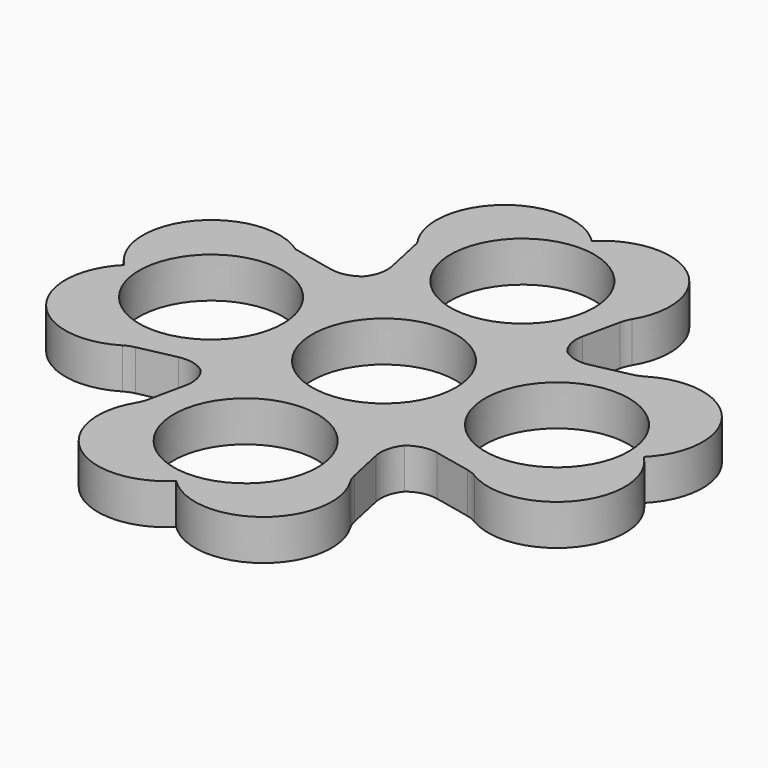
from build123d import *

# Parameters (mm, degrees)
F0_R        = 11.2522
F1_DEPTH    = 6.35
F2_T1_DEPTH = 6.35


# Not quite as in the source:
# - a fillet or chamfer that OpenCascade refuses, or shapes differently, is made with other operations: its cross-section is extruded or revolved along the edge and cut away or added


with BuildPart() as f1:
    # F0 (on Top) → F1 (new body)
    with BuildSketch(Plane.XY):
        with BuildLine():
            Line((-16.3332085084, 26.9033375639), (-14.2845390508, 17.386659874))
            ThreePointArc((-14.2845390508, 17.386659874), (-15.9113795359, 15.9113795359), (-17.386659874, 14.2845390508))
            Line((-17.386659874, 14.2845390508), (-26.9033375639, 16.3332085084))
            ThreePointArc((-26.9033375639, 16.3332085084), (-41.2837315607, 14.4844486959), (-40.64, 0))
            ThreePointArc((-40.64, 0), (-41.2837315607, -14.4844486959), (-26.9033375639, -16.3332085084))
            Line((-26.9033375639, -16.3332085084), (-17.386659874, -14.2845390508))
            ThreePointArc((-17.386659874, -14.2845390508), (-15.9113795359, -15.9113795359), (-14.2845390508, -17.386659874))
            Line((-14.2845390508, -17.386659874), (-16.3332085084, -26.9033375639))
            ThreePointArc((-16.3332085084, -26.9033375639), (-14.4844486959, -41.2837315607), (0, -40.64))
            ThreePointArc((0, -40.64), (14.4844486959, -41.2837315607), (16.3332085084, -26.9033375639))
            Line((16.3332085084, -26.9033375639), (14.2845390508, -17.386659874))
            ThreePointArc((14.2845390508, -17.386659874), (15.9113795359, -15.9113795359), (17.386659874, -14.2845390508))
            Line((17.386659874, -14.2845390508), (26.9033375639, -16.3332085084))
            ThreePointArc((26.9033375639, -16.3332085084), (41.2837315607, -14.4844486959), (40.64, 0))
            ThreePointArc((40.64, 0), (41.2837315607, 14.4844486959), (26.9033375639, 16.3332085084))
            Line((26.9033375639, 16.3332085084), (17.386659874, 14.2845390508))
            ThreePointArc((17.386659874, 14.2845390508), (15.9113795359, 15.9113795359), (14.2845390508, 17.386659874))
            Line((14.2845390508, 17.386659874), (16.3332085084, 26.9033375639))
            ThreePointArc((16.3332085084, 26.9033375639), (14.4844486959, 41.2837315607), (0, 40.64))
            ThreePointArc((0, 40.64), (-14.4844486959, 41.2837315607), (-16.3332085084, 26.9033375639))
        make_face()
        with Locations((0, -27.0631238818)):
            Circle(F0_R, mode=Mode.SUBTRACT)
        with Locations((-27.0631238818, 0)):
            Circle(F0_R, mode=Mode.SUBTRACT)
        Circle(F0_R, mode=Mode.SUBTRACT)
        with Locations((27.0631238818, 0)):
            Circle(F0_R, mode=Mode.SUBTRACT)
        with Locations((0, 27.0631238818)):
            Circle(F0_R, mode=Mode.SUBTRACT)
    extrude(amount=F1_DEPTH)

    # F2: fillet of radius 5.08 on 14 edges, made by hand

    # F2_s2 → F2_t1 (join)
    with BuildSketch(Plane.XY):
        with BuildLine():
            ThreePointArc((-15.61619491, 16.2011868084), (-17.7500326172, 14.9730442969), (-20.2107454114, 14.8924841735))
            Line((-20.2107454114, 14.8924841735), (-17.386659874, 14.2845390508))
            ThreePointArc((-17.386659874, 14.2845390508), (-16.5292313987, 15.2685463237), (-15.61619491, 16.2011868084))
        make_face()
        with BuildLine():
            ThreePointArc((-14.8924841735, 20.2107454114), (-14.9730442969, 17.7500326172), (-16.2011868084, 15.61619491))
            ThreePointArc((-16.2011868084, 15.61619491), (-15.2685463237, 16.5292313987), (-14.2845390508, 17.386659874))
            Line((-14.2845390508, 17.386659874), (-14.8924841735, 20.2107454114))
        make_face()
        with BuildLine():
            ThreePointArc((20.2107454114, -14.8924841735), (17.7500326172, -14.9730442969), (15.61619491, -16.2011868084))
            ThreePointArc((15.61619491, -16.2011868084), (16.5292313987, -15.2685463237), (17.386659874, -14.2845390508))
            Line((17.386659874, -14.2845390508), (20.2107454114, -14.8924841735))
        make_face()
        with BuildLine():
            ThreePointArc((25.9885821775, -16.1362877465), (26.7940259506, -16.3810221446), (27.5479957457, -16.7554071673))
            ThreePointArc((27.5479957457, -16.7554071673), (27.221867498, -16.5501087977), (26.9033375639, -16.3332085084))
            Line((26.9033375639, -16.3332085084), (25.9885821775, -16.1362877465))
        make_face()
        with BuildLine():
            ThreePointArc((27.5479957457, 16.7554071673), (26.7940259506, 16.3810221446), (25.9885821775, 16.1362877465))
            Line((25.9885821775, 16.1362877465), (26.9033375639, 16.3332085084))
            ThreePointArc((26.9033375639, 16.3332085084), (27.221867498, 16.5501087977), (27.5479957457, 16.7554071673))
        make_face()
        with BuildLine():
            ThreePointArc((20.2107454114, 14.8924841735), (17.7500326172, 14.9730442969), (15.61619491, 16.2011868084))
            ThreePointArc((15.61619491, 16.2011868084), (16.5292313987, 15.2685463237), (17.386659874, 14.2845390508))
            Line((17.386659874, 14.2845390508), (20.2107454114, 14.8924841735))
        make_face()
        with BuildLine():
            ThreePointArc((16.2011868084, 15.61619491), (14.9730442969, 17.7500326172), (14.8924841735, 20.2107454114))
            Line((14.8924841735, 20.2107454114), (14.2845390508, 17.386659874))
            ThreePointArc((14.2845390508, 17.386659874), (15.2685463237, 16.5292313987), (16.2011868084, 15.61619491))
        make_face()
        with BuildLine():
            ThreePointArc((16.1362877465, 25.9885821775), (16.3810221446, 26.7940259506), (16.7554071673, 27.5479957457))
            ThreePointArc((16.7554071673, 27.5479957457), (16.5501087977, 27.221867498), (16.3332085084, 26.9033375639))
            Line((16.3332085084, 26.9033375639), (16.1362877465, 25.9885821775))
        make_face()
        with BuildLine():
            ThreePointArc((-27.5479957457, -16.7554071673), (-26.7940259506, -16.3810221446), (-25.9885821775, -16.1362877465))
            Line((-25.9885821775, -16.1362877465), (-26.9033375639, -16.3332085084))
            ThreePointArc((-26.9033375639, -16.3332085084), (-27.221867498, -16.5501087977), (-27.5479957457, -16.7554071673))
        make_face()
        with BuildLine():
            ThreePointArc((-20.2107454114, -14.8924841735), (-17.7500326172, -14.9730442969), (-15.61619491, -16.2011868084))
            ThreePointArc((-15.61619491, -16.2011868084), (-16.5292313987, -15.2685463237), (-17.386659874, -14.2845390508))
            Line((-17.386659874, -14.2845390508), (-20.2107454114, -14.8924841735))
        make_face()
        with BuildLine():
            ThreePointArc((-16.2011868084, -15.61619491), (-14.9730442969, -17.7500326172), (-14.8924841735, -20.2107454114))
            Line((-14.8924841735, -20.2107454114), (-14.2845390508, -17.386659874))
            ThreePointArc((-14.2845390508, -17.386659874), (-15.2685463237, -16.5292313987), (-16.2011868084, -15.61619491))
        make_face()
        with BuildLine():
            ThreePointArc((-16.1362877465, -25.9885821775), (-16.3810221446, -26.7940259506), (-16.7554071673, -27.5479957457))
            ThreePointArc((-16.7554071673, -27.5479957457), (-16.5501087977, -27.221867498), (-16.3332085084, -26.9033375639))
            Line((-16.3332085084, -26.9033375639), (-16.1362877465, -25.9885821775))
        make_face()
        with BuildLine():
            ThreePointArc((16.7554071673, -27.5479957457), (16.3810221446, -26.7940259506), (16.1362877465, -25.9885821775))
            Line((16.1362877465, -25.9885821775), (16.3332085084, -26.9033375639))
            ThreePointArc((16.3332085084, -26.9033375639), (16.5501087977, -27.221867498), (16.7554071673, -27.5479957457))
        make_face()
        with BuildLine():
            ThreePointArc((14.8924841735, -20.2107454114), (14.9730442969, -17.7500326172), (16.2011868084, -15.61619491))
            ThreePointArc((16.2011868084, -15.61619491), (15.2685463237, -16.5292313987), (14.2845390508, -17.386659874))
            Line((14.2845390508, -17.386659874), (14.8924841735, -20.2107454114))
        make_face()
    extrude(amount=F2_T1_DEPTH)


solid = f1.part
